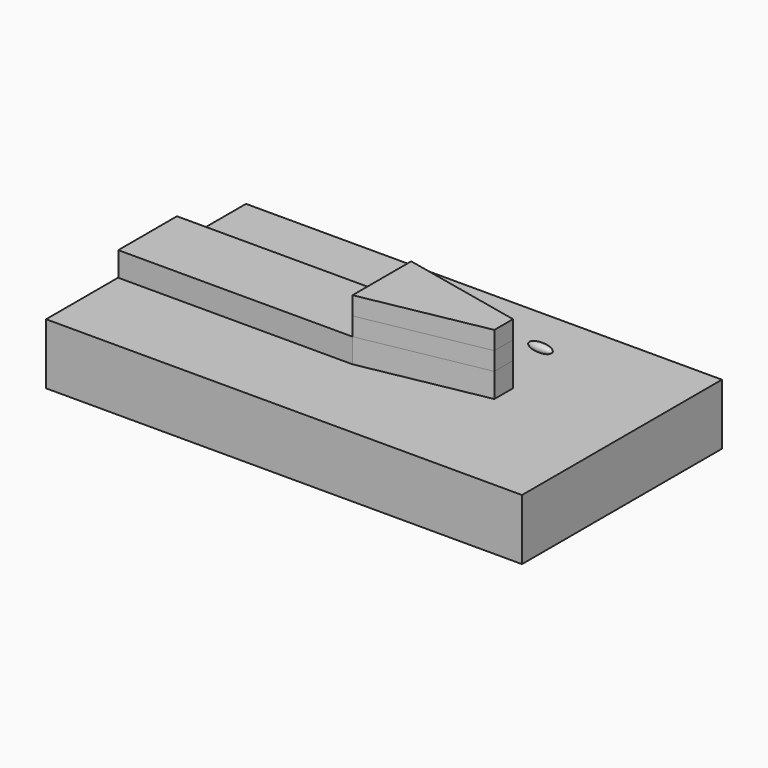
from build123d import *

# Parameters (mm, degrees)
F0_W     = 198.6827738583
F0_H     = 104.3191924691
F1_DEPTH = 25.4
F3_DEPTH = 10.16
F5_DEPTH = 7.62
F7_DEPTH = 7.62


# Not quite as in the source:
# - a feature names something its author has since deleted; it is built from what else it names


with BuildPart() as f1:
    # F0 (on Top) → F1 (new body)
    with BuildSketch(Plane.XY):
        with Locations((-49.9562527984, 0)):
            Rectangle(F0_W, F0_H)
    extrude(amount=-F1_DEPTH)


with BuildPart() as f3:
    # F2 (on face) → F3 (new body)
    with BuildSketch(Plane.XY):
        Polygon((0, 4.8675285652), (-51.4132715762, 16.0222817212), (-149.2118090391, 16.0222817212), (-149.2118090391, -14.602586627), (-51.4132715762, -14.602586627), (0, -4.8675285652), align=None)
    extrude(amount=F3_DEPTH)


with BuildPart() as f5:
    # F4 (on face) → F5 (new body)
    with BuildSketch(Plane.XY.offset(10.16)):
        Polygon((0, 4.8675285652), (-51.4132715762, 16.0222817212), (-51.4132715762, -14.602586627), (0, -4.8675285652), align=None)
    extrude(amount=F5_DEPTH)


with BuildPart() as f7:
    # F6 (on face) → F7 (new body)
    with BuildSketch(Plane.XY.offset(17.78)):
        Polygon((0, 4.8675285652), (-51.4132715762, 16.0222817212), (-51.4132715762, -14.602586627), (0, -4.8675285652), align=None)
    extrude(amount=F7_DEPTH)


with BuildPart() as f10:
    # F9 (on offset) → F10 (revolve)
    with BuildSketch(Plane.XY.offset(21.59)):
        with BuildLine():
            add(Edge.make_bspline(
                [(19.8862690043, 0.5098331603), (20.047106034, 2.2035256943), (15.0359997695, 2.2307201746), (10.024893505, 2.2579146549), (10.024893505, 0.5633492838)],
                knots=[3.1094951634, 3.1094951634, 3.1094951634, 4.6963402353, 4.6963402353, 6.2831853072, 6.2831853072, 6.2831853072], degree=2, weights=[1, 0.7014099885, 1, 0.7014099885, 1]))
            add(Edge.make_bspline(
                [(10.024893505, 0.5633492838), (10.024893505, 0.536584329), (10.027433859, 0.5098331603)],
                knots=[0, 0, 0, 0.0320974902, 0.0320974902, 0.0320974902], degree=2, weights=[1, 0.9998712217, 1]))
            Line((10.027433859, 0.5098331603), (19.8862690043, 0.5098331603))
        make_face()
    revolve(axis=Axis((15.8781609207, 0.5098331603, 21.59), (1, 0, 0)))


solid = Compound([f1.part, f3.part, f5.part, f7.part, f10.part])
